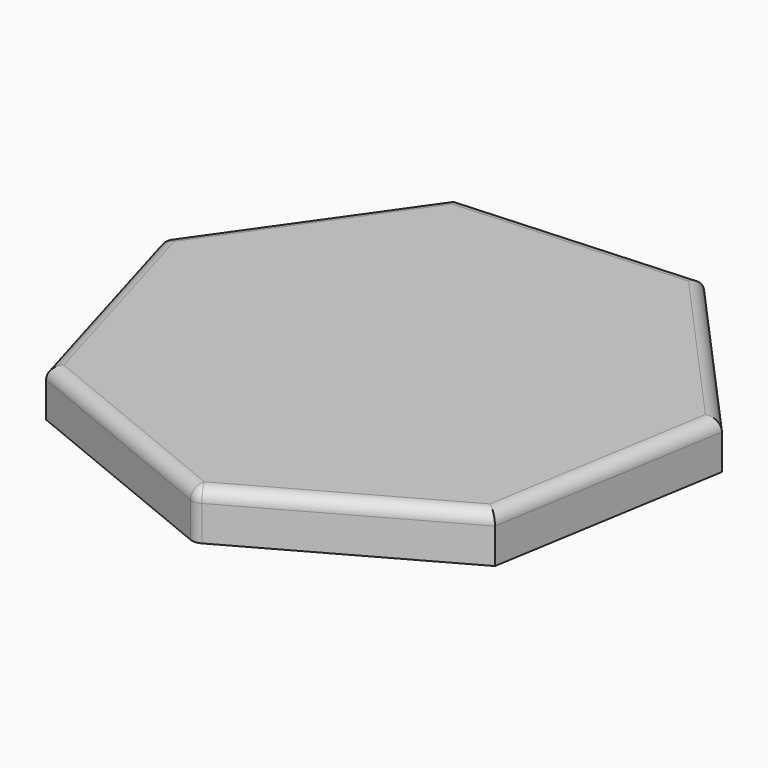
from build123d import *

# Parameters (mm, degrees)
F1_DEPTH     = 19
F2_R         = 5
F3_T1_DEPTH  = 104.8421979693
F3_T3_DEPTH  = 119.7500710634
F3_T5_DEPTH  = 119.7500710634
F3_T7_DEPTH  = 119.7500710634
F3_T9_DEPTH  = 104.8421979693
F3_T11_DEPTH = 20.0196827351
F3_T16_DEPTH = 5
F3_T22_DEPTH = 5


# Not quite as in the source:
# - a fillet or chamfer that OpenCascade refuses, or shapes differently, is made with other operations: its cross-section is extruded or revolved along the edge and cut away or added


with BuildPart() as f1:
    # F0 (on Top) → F1 (new body)
    with BuildSketch(Plane.XY):
        Polygon((41.3957443257, 101.0370281819), (-53.1841051002, 95.3600528356), (-107.7152386276, 17.8750127135), (-81.134600478, -73.0702765657), (6.5420466758, -108.9921572289), (89.2923992493, -62.8407204639), (104.8037539551, 30.6310605275), align=None)
    extrude(amount=F1_DEPTH)

    # F2
    f2_edges = [f1.edges().sort_by_distance(p)[0] for p in [
        (-94.42492, -27.597632, 19),
        (-37.296277, -91.031217, 19),
    ]]
    fillet(f2_edges, radius=F2_R)

    # F3: fillet of radius 5 on 7 edges, made by hand

    # F3_s2 → F3_t1 (cut)
    with BuildSketch(Plane(origin=(-39.2722507137, -21.9028770158, 0), x_dir=(0, 0, 1), z_dir=(0.8733539896, 0.4870860385, 0))):
        with BuildLine():
            ThreePointArc((19, 93.3752749449), (17.5355339059, 96.9108088508), (14, 98.3752749449))
            Line((14, 98.3752749449), (19, 98.3752749449))
            Line((19, 98.3752749449), (19, 93.3752749449))
        make_face()
    extrude(amount=F3_T1_DEPTH, mode=Mode.SUBTRACT)

    # F3_s4 → F3_t3 (cut)
    with BuildSketch(Plane(origin=(-9.8020286817, -59.067250771, 0), x_dir=(0, 0, 1), z_dir=(0.1637081063, 0.986508822, 0))):
        with BuildLine():
            ThreePointArc((19, 93.3752749449), (17.5355339059, 96.9108088508), (14, 98.3752749449))
            Line((14, 98.3752749449), (19, 98.3752749449))
            Line((19, 98.3752749449), (19, 93.3752749449))
        make_face()
    extrude(amount=F3_T3_DEPTH, mode=Mode.SUBTRACT)

    # F3_s6 → F3_t5 (cut)
    with BuildSketch(Plane(origin=(40.0691713151, -44.4913630949, 0), x_dir=(0, 0, 1), z_dir=(-0.66921332, 0.7430703414, 0))):
        with BuildLine():
            ThreePointArc((19, 93.3752749449), (17.5355339059, 96.9108088508), (14, 98.3752749449))
            Line((14, 98.3752749449), (19, 98.3752749449))
            Line((19, 98.3752749449), (19, 93.3752749449))
        make_face()
    extrude(amount=F3_T5_DEPTH, mode=Mode.SUBTRACT)

    # F3_s8 → F3_t7 (cut)
    with BuildSketch(Plane(origin=(59.7674680494, 3.58742845, 0), x_dir=(0, 0, 1), z_dir=(-0.9982034669, -0.0599152621, 0))):
        with BuildLine():
            ThreePointArc((19, 93.3752749449), (17.5355339059, 96.9108088508), (14, 98.3752749449))
            Line((14, 98.3752749449), (19, 98.3752749449))
            Line((19, 98.3752749449), (19, 93.3752749449))
        make_face()
    extrude(amount=F3_T7_DEPTH, mode=Mode.SUBTRACT)

    # F3_s10 → F3_t9 (cut)
    with BuildSketch(Plane(origin=(34.4596423084, 48.9648132019, 0), x_dir=(0, 0, 1), z_dir=(-0.5755260436, -0.8177834513, 0))):
        with BuildLine():
            ThreePointArc((14, 98.3752749449), (17.5355339059, 96.9108088508), (19, 93.3752749449))
            Line((19, 93.3752749449), (19, 98.3752749449))
            Line((19, 98.3752749449), (14, 98.3752749449))
        make_face()
    extrude(amount=F3_T9_DEPTH, mode=Mode.SUBTRACT)

    # F3_s12 → F3_t11 (cut)
    with BuildSketch(Plane.XY.offset(-6.0196827351)):
        with BuildLine():
            ThreePointArc((-106.3294449524, 19.8441314825), (-107.1730718062, 17.7850417962), (-107.0397478053, 15.5638301188))
            Line((-107.0397478053, 15.5638301188), (-107.7152386276, 17.8750127135))
            Line((-107.7152386276, 17.8750127135), (-106.3294449524, 19.8441314825))
        make_face()
        with BuildLine():
            ThreePointArc((4.3139297226, -108.0792784419), (6.5091183669, -108.443563249), (8.6449722488, -107.8193158622))
            Line((8.6449722488, -107.8193158622), (6.5420466758, -108.9921572289))
            Line((6.5420466758, -108.9921572289), (4.3139297226, -108.0792784419))
        make_face()
    extrude(amount=F3_T11_DEPTH, mode=Mode.SUBTRACT)


with BuildPart() as f3_tool14:
    # F3_s15 → F3_t16 (new body)
    with BuildSketch(Plane.XY.offset(14)):
        Polygon((6.2095420561, -103.4525459145), (4.3139297226, -108.0792784419), (6.5420466758, -108.9921572289), (8.6449722488, -107.8193158622), align=None)
    extrude(amount=F3_T16_DEPTH)

    # F3_s17 → F3_t18 (revolve, cut)
    with BuildSketch(Plane(origin=(6.2095420561, -103.4525459145, 14), x_dir=(-0.0599152621, 0.9982034669, 0), z_dir=(0.9982034669, 0.0599152621, 0))):
        with BuildLine():
            ThreePointArc((0, -5), (5, 0), (0, 5))
            Line((0, 5), (0, -5))
        make_face()
    revolve(axis=Axis((6.2095420561, -103.4525459145, 14), (0, 0, 1)), mode=Mode.SUBTRACT)


with BuildPart() as f1_1:
    add(f1.part)

    # F3_t13: cut F3_tool14
    add(f3_tool14.part, mode=Mode.SUBTRACT)


with BuildPart() as f3_tool20:
    # F3_s21 → F3_t22 (new body)
    with BuildSketch(Plane.XY.offset(14)):
        Polygon((-102.240527696, 16.9665012646), (-106.3294449524, 19.8441314825), (-107.7152386276, 17.8750127135), (-107.0397478053, 15.5638301188), align=None)
    extrude(amount=F3_T22_DEPTH)

    # F3_s23 → F3_t24 (revolve, cut)
    with BuildSketch(Plane(origin=(-102.240527696, 16.9665012646, 14), x_dir=(0.986508822, -0.1637081063, 0), z_dir=(-0.1637081063, -0.986508822, 0))):
        with BuildLine():
            ThreePointArc((0, -5), (5, 0), (0, 5))
            Line((0, 5), (0, -5))
        make_face()
    revolve(axis=Axis((-102.240527696, 16.9665012646, 14), (0, 0, 1)), mode=Mode.SUBTRACT)


with BuildPart() as f1_2:
    add(f1_1.part)

    # F3_t19: cut F3_tool20
    add(f3_tool20.part, mode=Mode.SUBTRACT)


solid = f1_2.part
